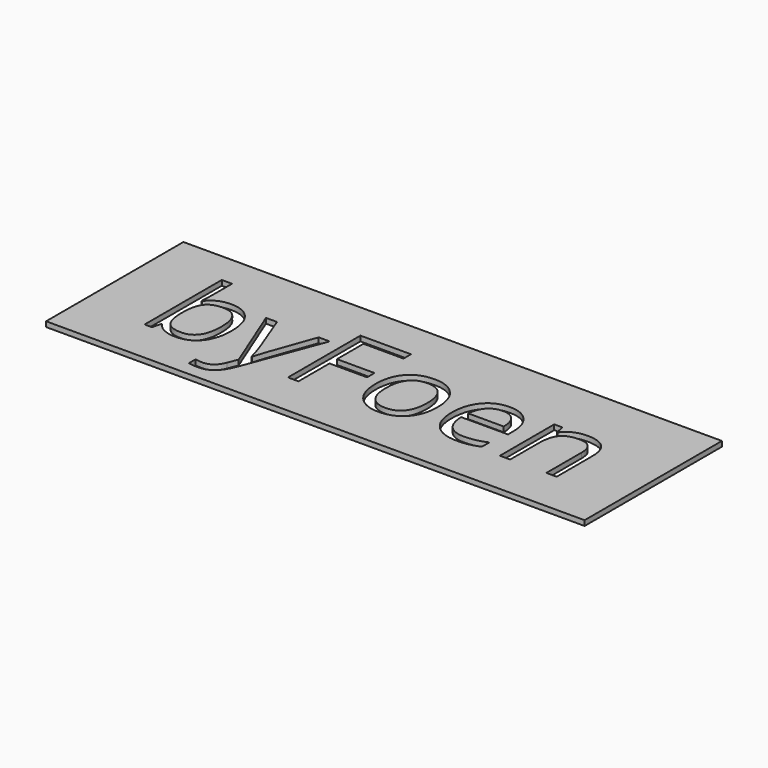
from build123d import *

# Parameters (mm, degrees)
F0_W         = 126.1567175388
F0_H         = 40.2184426785
F1_DEPTH     = 1.2
F2_TEXT_SIZE = 29.7470988395
F3_DEPTH     = 1.201


# Not quite as in the source:
# - Text() gives the source's letters only with a copy of the font that has no kerning and outlines rounded to 1/6400 em; it was checked with that copy


with BuildPart() as f1:
    # F0 (on Top) → F1 (new body)
    with BuildSketch(Plane.XY):
        Rectangle(F0_W, F0_H)
    extrude(amount=F1_DEPTH)

    # F2 (on face) → F3 (cut, through all)
    with BuildSketch(Plane.XY.offset(1.2)):
        with Locations((-50.7651865482, -9.8515907302)):
            Text('byFoen', F2_TEXT_SIZE, font='Open Sans', text_align=(TextAlign.LEFT, TextAlign.BOTTOM))
    extrude(amount=-F3_DEPTH, mode=Mode.SUBTRACT)


solid = f1.part
